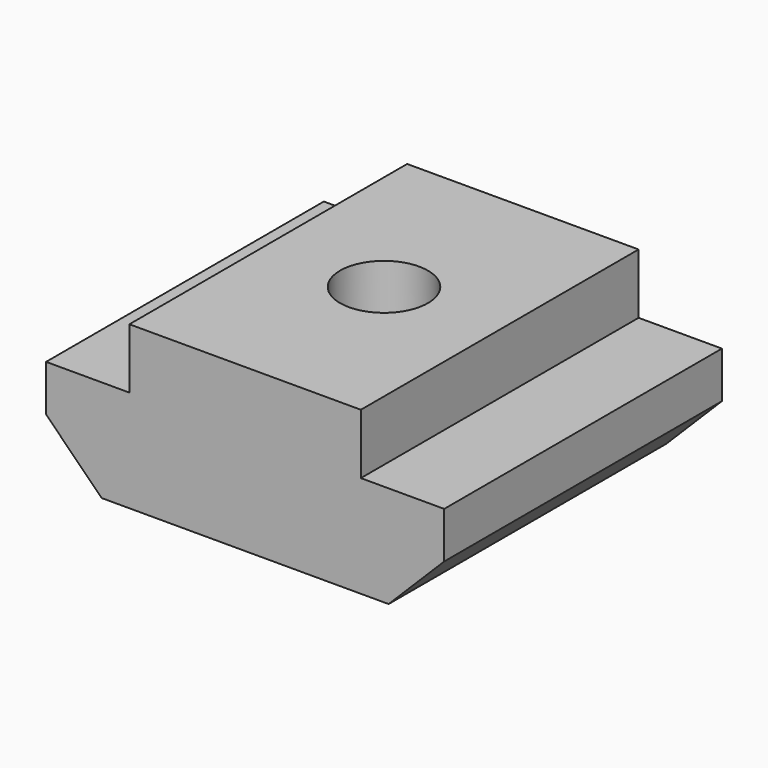
from build123d import *

# Parameters (mm, degrees)
F1_DEPTH = 15
F3_D     = 3.8
F4_R     = 1.9
F5_DEPTH = 2.7


with BuildPart() as f1:
    # F0 (on Front) → F1 (new body)
    with BuildSketch(Plane.XZ):
        Polygon((0, 7), (0, 0), (6.2, 0), (8.6, 2.4), (8.6, 4.4), (5, 4.4), (5, 7), align=None)
        Polygon((-8.6, 4.4), (-8.6, 2.4), (-6.2, 0), (0, 0), (0, 7), (-5, 7), (-5, 4.4), align=None)
    extrude(amount=F1_DEPTH)

    # F3 (through all)
    with Locations(Plane.XY.offset(7)):
        with Locations((0, -7.5)):
            Hole(F3_D / 2)

    # F4 (on face) → F5 (cut)
    with BuildSketch(Plane(origin=(0, 0, 0), x_dir=(1, 0, 0), z_dir=(0, 0, -1))):
        Polygon((-3, 5.7679491924), (0, 4.0358983849), (3, 5.7679491924), (3, 9.2320508076), (0, 10.9641016151), (-3, 9.2320508076), align=None)
        with Locations((0, 7.5)):
            Circle(F4_R, mode=Mode.SUBTRACT)
    extrude(amount=-F5_DEPTH, mode=Mode.SUBTRACT)


solid = f1.part
